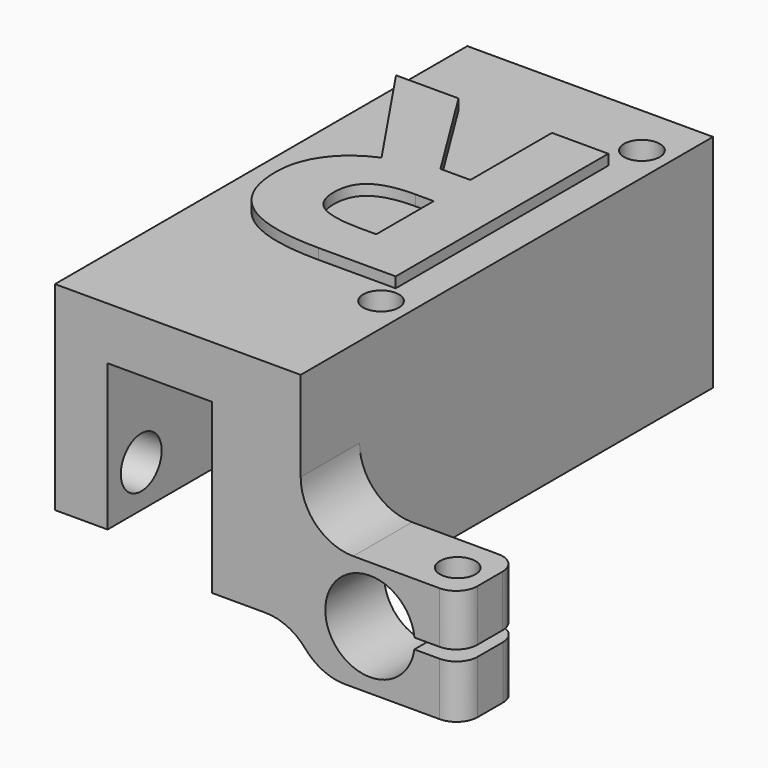
from build123d import *

# Parameters (mm, degrees)
F1_DEPTH      = 7
F2_DEPTH      = 42
F3_R          = 1.7
F3_R_2        = 11
F4_DEPTH      = 21.001
F5_R          = 4.25
F6_DEPTH      = 10
F7_DEPTH      = 21.001
F8_R          = 1.4
F9_DEPTH      = 11.017224352
F8_R_2        = 1.7
F10_DEPTH     = 4.9107017738
F11_R         = 5
F12_R         = 5
F13_R         = 5
F14_R         = 2
F15_R         = 2.2
F15_R_2       = 2.4255023423
F16_DEPTH     = 6
F17_TEXT_SIZE = 35.3857979109
F18_DEPTH     = 1


# Not quite as in the source:
# - a feature names something its author has since deleted; it is built from what else it names
# - Text() gives the source's letters only with a copy of the font that has no kerning and outlines rounded to 1/6400 em; it was checked with that copy


with BuildPart() as f1:
    # F0 (on Front) → F1 (new body)
    with BuildSketch(Plane.XZ):
        Polygon((-18.6721007523, 29.8099789735), (-18.6721007523, 10.8925135386), (-13.6721007523, 10.8925135386), (-13.6721007523, 24.8099789735), (-3.7221007523, 24.8099789735), (-3.7221007523, 8.8099789735), (4.6880548998, 8.8099789735), (4.6880548998, 16.2656020473), (4.6880548998, 29.8099789735), align=None)
        Polygon((19.8763195603, 16.2417280634), (4.6880548998, 16.2656020473), (4.6880548998, 8.8099789735), (6.1033044869, 5.2860832236), (19.9053367778, 5.2860832236), (19.9053367778, 10.343908232), (13.2360510706, 10.343908232), (13.2360510706, 11.3388913612), (19.8763195603, 11.3388913612), align=None)
    extrude(amount=F1_DEPTH)

    # F0 (on Front) → F2 (join)
    with BuildSketch(Plane.XZ):
        Polygon((-18.6721007523, 29.8099789735), (-18.6721007523, 10.8925135386), (-13.6721007523, 10.8925135386), (-13.6721007523, 24.8099789735), (-3.7221007523, 24.8099789735), (-3.7221007523, 8.8099789735), (4.6880548998, 8.8099789735), (4.6880548998, 16.2656020473), (4.6880548998, 29.8099789735), align=None)
    extrude(amount=-F2_DEPTH)

    # F3 (on face) → F4 (cut, through all)
    with BuildSketch(Plane(origin=(0, 0, 8.8099789735), x_dir=(1, 0, 0), z_dir=(0, 0, -1))):
        with Locations((1.9280548998, -6)):
            Circle(F3_R)
        with Locations((1.9280548998, -37)):
            Circle(F3_R)
        with Locations((17.4280548998, -21.5)):
            Circle(F3_R_2)
    extrude(amount=-F4_DEPTH, mode=Mode.SUBTRACT)

    # F5 (on face) → F6 (cut)
    with BuildSketch(Plane.XZ.offset(7)):
        with Locations((11.2778992477, 10.8989789735)):
            Circle(F5_R)
    extrude(amount=-F6_DEPTH, mode=Mode.SUBTRACT)

    # F3 (on face) → F7 (cut, through all)
    with BuildSketch(Plane(origin=(0, 0, 8.8099789735), x_dir=(1, 0, 0), z_dir=(0, 0, -1))):
        with Locations((1.9280548998, -6)):
            Circle(F3_R)
        with Locations((1.9280548998, -37)):
            Circle(F3_R)
        with Locations((17.4280548998, -21.5)):
            Circle(F3_R_2)
    extrude(amount=-F7_DEPTH, mode=Mode.SUBTRACT)

    # F8 (on face) → F9 (cut, through all)
    with BuildSketch(Plane(origin=(0.0255789386, 0, 16.2729308554), x_dir=(0.9999987646, 0, -0.0015718685), z_dir=(0.0015718685, 0, 0.9999987646))):
        with Locations((16.850765145, -3.5767070949)):
            Circle(F8_R)
    extrude(amount=-F9_DEPTH, mode=Mode.SUBTRACT)

    # F8 (on face) → F10 (cut, through all)
    with BuildSketch(Plane(origin=(0.0255789386, 0, 16.2729308554), x_dir=(0.9999987646, 0, -0.0015718685), z_dir=(0.0015718685, 0, 0.9999987646))):
        with Locations((16.850765145, -3.5767070949)):
            Circle(F8_R_2)
        with Locations((16.850765145, -3.5767070949)):
            Circle(F8_R, mode=Mode.SUBTRACT)
    extrude(amount=-F10_DEPTH, mode=Mode.SUBTRACT)

    # F11
    f11_edges = [f1.edges().sort_by_distance(p)[0] for p in [
        (4.688055, -3.5, 16.265602),
    ]]
    fillet(f11_edges, radius=F11_R)

    # F12
    f12_edges = [f1.edges().sort_by_distance(p)[0] for p in [
        (4.688055, -3.5, 8.809979),
    ]]
    fillet(f12_edges, radius=F12_R)

    # F13
    f13_edges = [f1.edges().sort_by_distance(p)[0] for p in [
        (6.103304, -3.5, 5.286083),
    ]]
    fillet(f13_edges, radius=F13_R)

    # F14
    f14_edges = [f1.edges().sort_by_distance(p)[0] for p in [
        (19.87632, -7, 13.79031),
        (19.905337, -7, 7.814996),
        (19.87632, 0, 13.79031),
        (19.905337, 0, 7.814996),
    ]]
    fillet(f14_edges, radius=F14_R)

    # F15 (on face) → F16 (cut)
    with BuildSketch(Plane(origin=(-18.6721007523, 0, 0), x_dir=(0, -1, 0), z_dir=(-1, 0, 0))):
        with Locations((-38, 14.8925135386)):
            Circle(F15_R)
        with Locations((3, 14.8925135386)):
            Circle(F15_R_2)
    extrude(amount=-F16_DEPTH, mode=Mode.SUBTRACT)

    # F17 (on face) → F18 (join)
    with BuildSketch(Plane.XY.offset(29.8099789735)):
        with Locations(Location((4.6880548998, 33.5274108189), (0, 0, 180))):
            Text('R', F17_TEXT_SIZE, font='Open Sans', font_style=FontStyle.BOLD, text_align=(TextAlign.LEFT, TextAlign.BOTTOM))
    extrude(amount=F18_DEPTH)


solid = f1.part
